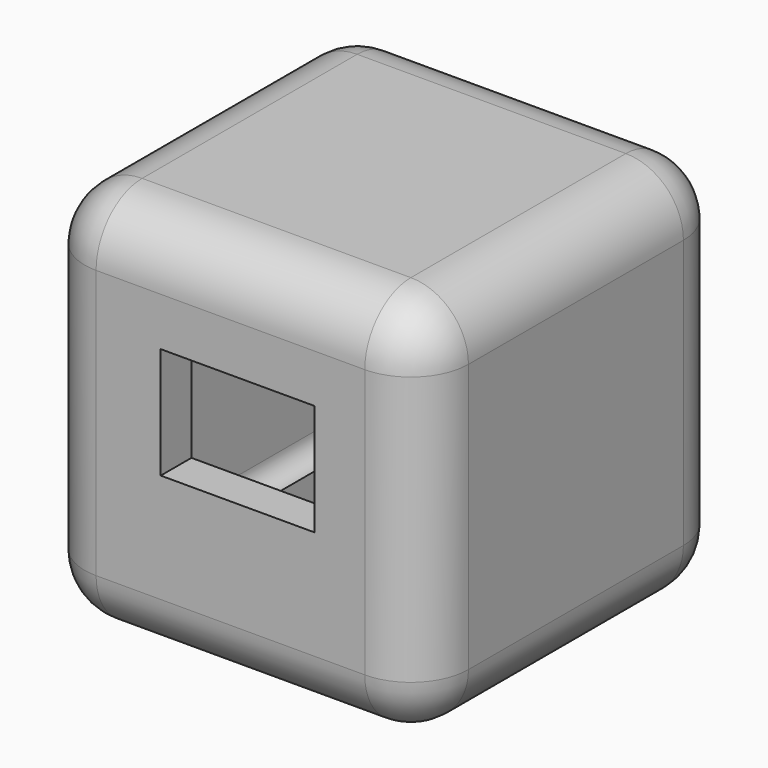
from build123d import *

# Parameters (mm, degrees)
F0_W     = 1000
F0_H     = 1000
F1_DEPTH = 1000
F2_R     = 150
F3_W     = 400
F3_H     = 290
F4_DEPTH = 500
F5_T     = 100
F6_W     = 700
F6_H     = 700
F7_DEPTH = 500


# Not quite as in the source:
# - a shell that OpenCascade refuses in one call is made with other operations: the cavity is built on its own and cut out


with BuildPart() as f1:
    # F0 (on Front) → F1 (new body)
    with BuildSketch(Plane.XZ):
        with Locations((181.6326389278, 340.3687052429)):
            Rectangle(F0_W, F0_H)
    extrude(amount=F1_DEPTH)

    # F2
    f2_edges = [f1.edges().sort_by_distance(p)[0] for p in [
        (181.632639, -1000, 840.368705),
        (681.632639, -500, 840.368705),
        (681.632639, -1000, 340.368705),
        (-318.367361, -1000, 340.368705),
        (-318.367361, -500, 840.368705),
        (181.632639, 0, 840.368705),
        (681.632639, 0, 340.368705),
        (-318.367361, 0, 340.368705),
        (181.632639, -1000, -159.631295),
        (681.632639, -500, -159.631295),
        (-318.367361, -500, -159.631295),
        (181.632639, 0, -159.631295),
    ]]
    fillet(f2_edges, radius=F2_R)

    # F3 (on face) → F4 (cut)
    with BuildSketch(Plane.XZ.offset(1000)):
        with Locations((200, 419.5188772678)):
            Rectangle(F3_W, F3_H)
    extrude(amount=-F4_DEPTH, mode=Mode.SUBTRACT)

    # F5: shell of thickness 100, made by hand


with BuildPart() as f5_core1:
    # F5_t2: copy of F1
    add(f1.part)

    # the walls: a layer under each face that stays
    f5_faces = [f5_core1.faces().sort_by_distance(p)[0] for p in [
        (-318.3673610722, -500, 340.3687052429),
        (-274.4333782502, -956.066017178, 340.3687052429),
        (-274.4333782502, -500, 796.4347224209),
        (-274.4333782502, -500, -115.6973119351),
        (-274.4333782502, -43.933982822, 340.3687052429),
        (-274.4333782502, -925, 765.3687052429),
        (-51.7006944055, -1000, 107.0353719095),
        (-243.3673610722, -925, -115.6973119351),
        (-243.3673610722, -43.933982822, 765.3687052429),
        (181.6326389278, -500, 840.3687052429),
        (-243.3673610722, -75, -115.6973119351),
        (181.6326389278, -500, -159.6312947571),
        (181.6326389278, 0, 340.3687052429),
        (181.6326389278, -956.066017178, 796.4347224209),
        (637.6986561058, -956.066017178, 340.3687052429),
        (181.6326389278, -956.066017178, -115.6973119351),
        (200, -750, 564.5188772678),
        (181.6326389278, -43.933982822, 796.4347224209),
        (637.6986561058, -500, 796.4347224209),
        (181.6326389278, -43.933982822, -115.6973119351),
        (637.6986561058, -500, -115.6973119351),
        (637.6986561058, -43.933982822, 340.3687052429),
        (637.6986561058, -925, 765.3687052429),
        (681.6326389278, -500, 340.3687052429),
        (606.6326389278, -925, -115.6973119351),
        (606.6326389278, -43.933982822, 765.3687052429),
        (606.6326389278, -75, -115.6973119351),
    ]]
    thicken(f5_faces, amount=-F5_T, mode=Mode.SUBTRACT)


with BuildPart() as f1_1:
    add(f1.part)

    # what is left inside the walls is the cavity
    f5_cavity = [f5_core1.part.solids().sort_by_distance(p)[0] for p in [
        (181.632639, -101, 223.702039),
    ]]
    add(f5_cavity, mode=Mode.SUBTRACT)

    # F6 (on face) → F7 (cut)
    with BuildSketch(Plane(origin=(0, 0, -159.6312947571), x_dir=(1, 0, 0), z_dir=(0, 0, -1))):
        with Locations((181.6326389278, 500)):
            Rectangle(F6_W, F6_H)
    extrude(amount=-F7_DEPTH, mode=Mode.SUBTRACT)


solid = f1_1.part
